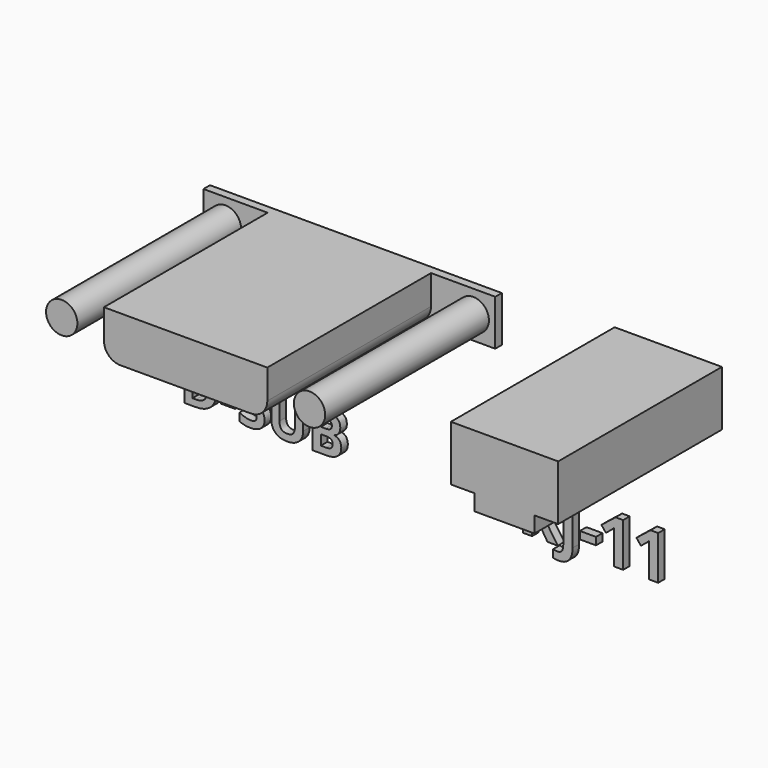
from build123d import *

# Parameters (mm, degrees)
F4_TEXT_SIZE = 13.2338557806
F6_DEPTH     = 2
F5_TEXT_SIZE = 14.9878673255
F7_DEPTH     = 2
F8_DEPTH     = 25
F2_R         = 3.8262968701
F10_DEPTH    = 25
F13_DEPTH    = 2


# Not quite as in the source:
# - a feature names something its author has since deleted; it is built from what else it names
# - Text() gives the source's letters only with a copy of the font that has no kerning and outlines rounded to 1/6400 em; it was checked with that copy


with BuildPart() as f6:
    # F4 (on offset) → F6 (new body)
    with BuildSketch(Plane.XZ):
        with Locations((-209.4969600439, 69.5083737373)):
            Text('D-SUB', F4_TEXT_SIZE, font='Open Sans', font_style=FontStyle.BOLD, text_align=(TextAlign.LEFT, TextAlign.BOTTOM))
    extrude(amount=F6_DEPTH)


with BuildPart() as f7:
    # F5 (on offset) → F7 (new body)
    with BuildSketch(Plane.XZ):
        with Locations((-126.9602179527, 68.4673115611)):
            Text('RJ-11', F5_TEXT_SIZE, font='Open Sans', font_style=FontStyle.BOLD, text_align=(TextAlign.LEFT, TextAlign.BOTTOM))
    extrude(amount=F7_DEPTH)


with BuildPart() as f8:
    # F3 (on offset) → F8 (new body)
    with BuildSketch(Plane.XZ):
        Polygon((-98.5648352653, 101.9628383219), (-111.6722151637, 101.9628383219), (-124.7795950621, 101.9628383219), (-124.7795950621, 88.4740743786), (-118.9821027219, 88.4740743786), (-118.9821027219, 84.5703594387), (-111.6722151637, 84.5703594387), (-104.3623276055, 84.5703594387), (-104.3623276055, 88.4740743786), (-98.5648352653, 88.4740743786), align=None)
    extrude(amount=-F8_DEPTH)

    # F9: F8 across face


with BuildPart() as f8_1:
    add(f8.part)
    add(f8.part.mirror(Plane(origin=(-111.6722151637, 0, 94.0099448002), x_dir=(1, 0, 0), z_dir=(0, -1, 0))))


with BuildPart() as f10:
    # F2 (on Front) → F10 (new body)
    with BuildSketch(Plane.XZ):
        with Locations((-219.8419403285, 93.4452861547)):
            Circle(F2_R)
    extrude(amount=-F10_DEPTH)



with BuildPart() as f10b:
    # F2 (on Front) → F10, piece 2 (new body)
    with BuildSketch(Plane.XZ):
        with BuildLine():
            Line((-169.621844776, 99.0324653685), (-209.5302743837, 99.0324653685))
            Line((-209.5302743837, 99.0324653685), (-209.5302743837, 91.858106941))
            ThreePointArc((-209.5302743837, 91.858106941), (-208.3587015085, 89.0296798162), (-205.5302743837, 87.858106941))
            Line((-205.5302743837, 87.858106941), (-173.621844776, 87.858106941))
            ThreePointArc((-173.621844776, 87.858106941), (-170.7934176512, 89.0296798162), (-169.621844776, 91.858106941))
            Line((-169.621844776, 91.858106941), (-169.621844776, 99.0324653685))
        make_face()
    extrude(amount=-F10_DEPTH)


with BuildPart() as f10c:
    # F2 (on Front) → F10, piece 3 (new body)
    with BuildSketch(Plane.XZ):
        with Locations((-159.3101788312, 93.4452861547)):
            Circle(F2_R)
    extrude(amount=-F10_DEPTH)


with BuildPart() as f10_1:
    add(f10.part)

    add(f10b.part)  # F11 merges F10b

    add(f10c.part)  # F11 merges F10c
    # F11: F10c, F10b, F10 across face
    add(f10c.part.mirror(Plane(origin=(-189.5760595798, 0, 93.5186956063), x_dir=(1, 0, 0), z_dir=(0, -1, 0))))
    add(f10b.part.mirror(Plane(origin=(-189.5760595798, 0, 93.5186956063), x_dir=(1, 0, 0), z_dir=(0, -1, 0))))
    add(f10.part.mirror(Plane(origin=(-189.5760595798, 0, 93.5186956063), x_dir=(1, 0, 0), z_dir=(0, -1, 0))))

    # F12 (on face) → F13 (join)
    with BuildSketch(Plane(origin=(0, 25, 0), x_dir=(-1, 0, 0), z_dir=(0, 1, 0))):
        with BuildLine():
            Line((209.5302743837, 91.858106941), (209.5302743837, 99.0324653685))
            Line((209.5302743837, 99.0324653685), (169.621844776, 99.0324653685))
            Line((169.621844776, 99.0324653685), (169.621844776, 91.858106941))
            ThreePointArc((169.621844776, 91.858106941), (170.7934176512, 89.0296798162), (173.621844776, 87.858106941))
            Line((173.621844776, 87.858106941), (205.5302743837, 87.858106941))
            ThreePointArc((205.5302743837, 87.858106941), (208.3587015085, 89.0296798162), (209.5302743837, 91.858106941))
        make_face()
        with BuildLine():
            Line((225.2146303654, 99.0324653685), (209.5302743837, 99.0324653685))
            Line((209.5302743837, 99.0324653685), (209.5302743837, 91.858106941))
            ThreePointArc((209.5302743837, 91.858106941), (208.3587015085, 89.0296798162), (205.5302743837, 87.858106941))
            Line((205.5302743837, 87.858106941), (225.2146303654, 87.858106941))
            Line((225.2146303654, 87.858106941), (225.2146303654, 99.0324653685))
        make_face()
        with BuildLine():
            Line((169.621844776, 91.858106941), (169.621844776, 99.0324653685))
            Line((169.621844776, 99.0324653685), (153.9374887943, 99.0324653685))
            Line((153.9374887943, 99.0324653685), (153.9374887943, 87.858106941))
            Line((153.9374887943, 87.858106941), (173.621844776, 87.858106941))
            ThreePointArc((173.621844776, 87.858106941), (170.7934176512, 89.0296798162), (169.621844776, 91.858106941))
        make_face()
    extrude(amount=F13_DEPTH)


solid = Compound([f6.part, f7.part, f8_1.part, f10_1.part])
